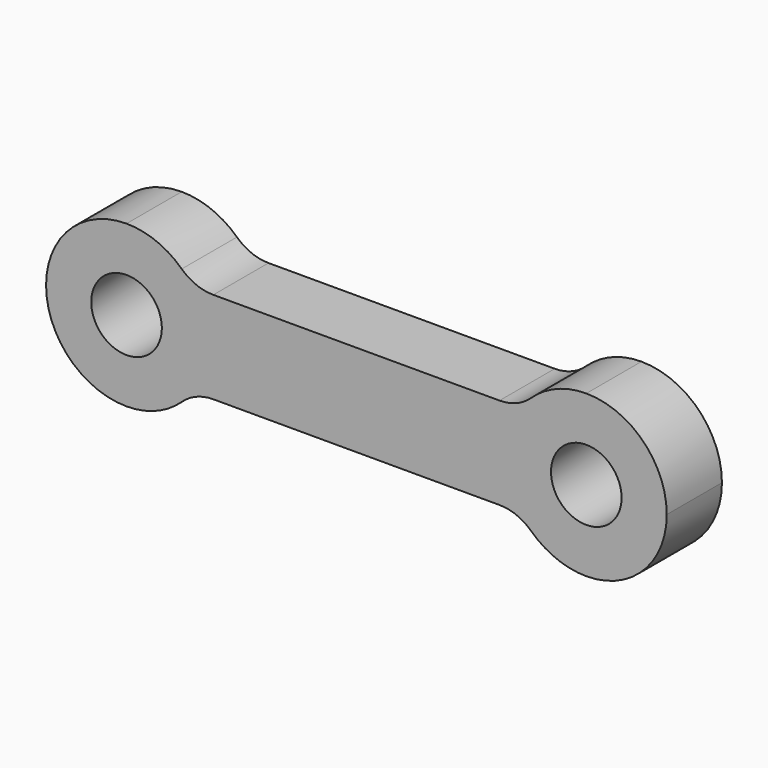
from build123d import *

# Parameters (mm, degrees)
F0_W     = 21.43125
F0_H     = 2.38125
F1_DEPTH = 5.55625
F2_R     = 2.778115
F3_R     = 1.2192
F4_DEPTH = 25.4


# Not quite as in the source:
# - a fillet or chamfer is up to 0.001 mm smaller than in the source, because OpenCascade refuses the exact size
# - ends of sketch curves that miss each other by under 0.0002 mm in the source are joined


with BuildPart() as f1:
    # F0 (on Top) → F1 (new body)
    with BuildSketch(Plane.XY):
        with Locations((16.6664377481, 21.9699217558)):
            Rectangle(F0_W, F0_H)
    extrude(amount=F1_DEPTH)

    # F2 (radius 2.778125 in the source; OpenCascade refuses exactly that, so slightly less here)
    f2_edges = [f1.edges().sort_by_distance(p)[0] for p in [
        (27.382063, 21.969922, 5.55625),
        (27.382063, 21.969922, 0),
        (5.950813, 21.969922, 5.55625),
        (5.950813, 21.969922, 0),
    ]]
    fillet(f2_edges, radius=F2_R)

    # F3 (on face) → F4 (cut)
    with BuildSketch(Plane.XZ.offset(-20.7792967558)):
        with Locations((8.7289377481, 2.778125)):
            Circle(F3_R)
        with Locations((24.6039377481, 2.778125)):
            Circle(F3_R)
        with BuildLine():
            Line((24.6039477481, 5.55625), (8.7289277481, 5.55625))
            ThreePointArc((8.7289277481, 5.55625), (9.7548283932, 5.3598931731), (10.6356999108, 4.7985795455))
            ThreePointArc((10.6356999108, 4.7985795455), (11.1390550638, 4.4778289011), (11.7252782896, 4.365625))
            Line((11.7252782896, 4.365625), (21.6075972066, 4.365625))
            ThreePointArc((21.6075972066, 4.365625), (22.1938204324, 4.4778289011), (22.6971755853, 4.7985795455))
            ThreePointArc((22.6971755853, 4.7985795455), (23.5780471029, 5.3598931731), (24.6039477481, 5.55625))
        make_face()
        with BuildLine():
            ThreePointArc((10.6356999108, 0.7576704545), (9.7548283932, 0.1963568269), (8.7289377481, 0))
            Line((8.7289377481, 0), (24.6039477481, 0))
            ThreePointArc((24.6039477481, 0), (23.5780471029, 0.1963568269), (22.6971755853, 0.7576704545))
            ThreePointArc((22.6971755853, 0.7576704545), (22.1938204324, 1.0784210989), (21.6075972066, 1.190625))
            Line((21.6075972066, 1.190625), (11.7252782896, 1.190625))
            ThreePointArc((11.7252782896, 1.190625), (11.1390550638, 1.0784210989), (10.6356999108, 0.7576704545))
        make_face()
    extrude(amount=-F4_DEPTH, mode=Mode.SUBTRACT)


solid = f1.part
